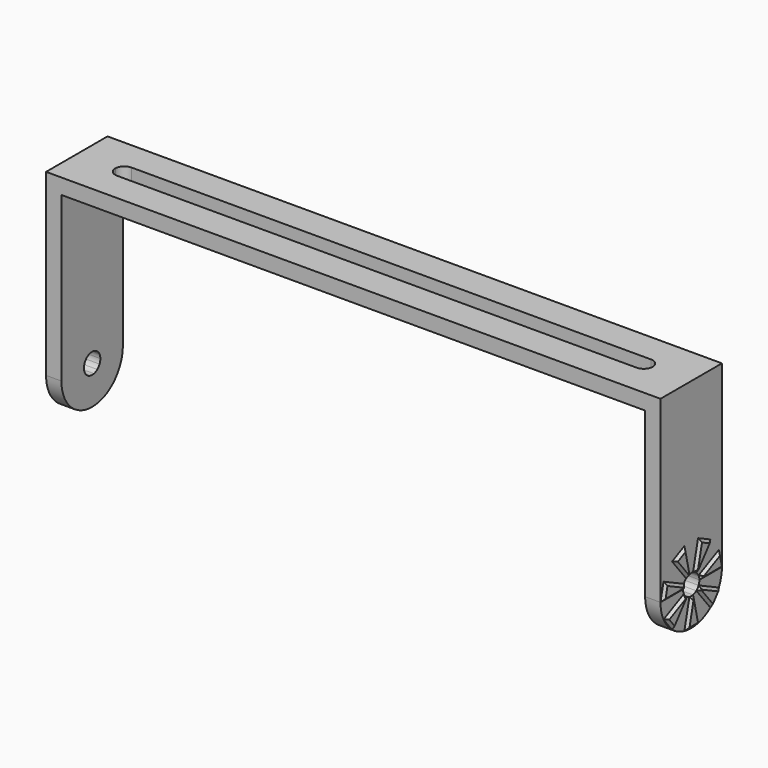
from build123d import *

# Parameters (mm, degrees)
F0_W                     = 3
F0_H                     = 15
F1_DEPTH                 = 35
F2_DEPTH                 = 3
F3_W                     = 3
F3_H                     = 7.5
F6_DEPTH                 = 0.5
DRAFT_F6_DRAFTED_ANGLE   = 45
DRAFT_F6_2_DRAFTED_ANGLE = 45
DRAFT_F6_3_DRAFTED_ANGLE = 45
DRAFT_F6_4_DRAFTED_ANGLE = 45
DRAFT_F6_5_DRAFTED_ANGLE = 45
DRAFT_F6_6_DRAFTED_ANGLE = 45
DRAFT_F6_7_DRAFTED_ANGLE = 45
F7_DEPTH                 = 25


# Not quite as in the source:
# - an extrude with a draft is written as a straight extrude whose walls are then drafted


with BuildPart() as f1:
    # F0 (on Top) → F1 (new body)
    with BuildSketch(Plane.XY):
        with Locations((-58.5, 0)):
            Rectangle(F0_W, F0_H)
    extrude(amount=-F1_DEPTH)

    # F0 (on Top) → F2 (join)
    with BuildSketch(Plane.XY):
        with BuildLine():
            Line((0, 1.75), (0, 7.5))
            Line((0, 7.5), (-57, 7.5))
            Line((-57, 7.5), (-57, -7.5))
            Line((-57, -7.5), (0, -7.5))
            Line((0, -7.5), (0, -1.75))
            Line((0, -1.75), (-50.7319065422, -1.75))
            ThreePointArc((-50.7319065422, -1.75), (-51.9693434093, -1.2374368671), (-52.4819065422, 0))
            ThreePointArc((-52.4819065422, 0), (-51.9693434093, 1.2374368671), (-50.7319065422, 1.75))
            Line((-50.7319065422, 1.75), (0, 1.75))
        make_face()
    extrude(amount=-F2_DEPTH)

    # F3 (on face) → F4 (revolve)
    with BuildSketch(Plane(origin=(0, 0, -35), x_dir=(1, 0, 0), z_dir=(0, 0, -1))):
        with Locations((-58.5, 3.75)):
            Rectangle(F3_W, F3_H)
    revolve(axis=Axis((-54.6439792961, 0, -35), (1, 0, 0)))


with BuildPart() as f6_drafted:
    # F5 (on face) → F6 (new body)
    with BuildSketch(Plane(origin=(-60, 0, 0), x_dir=(0, -1, 0), z_dir=(-1, 0, 0))):
        with BuildLine():
            Line((4.6761735139, -40.8637361185), (6.7572665093, -38.2541280434))
            Line((6.7572665093, -38.2541280434), (1.8019377358, -35.8677674782))
            ThreePointArc((1.8019377358, -35.8677674782), (1.5636629649, -36.2469796037), (1.2469796037, -36.5636629649))
            Line((1.2469796037, -36.5636629649), (4.6761735139, -40.8637361185))
        make_face()
    extrude(amount=F6_DEPTH)

    # draft_F6_drafted
    draft_f6_drafted_walls = [f6_drafted.faces().sort_by_distance(p)[0] for p in [
        (-60.3333333333, -1.5636629649, -36.2469796037),
        (-60.3333333333, -2.9615765588, -38.7136995417),
        (-60.3333333333, -5.7167200116, -39.5589320809),
        (-60.3333333333, -4.2796021225, -37.0609477608),
    ]]
    draft(draft_f6_drafted_walls, neutral_plane=Plane(origin=(-60, 0, 0), x_dir=(0, -1, 0), z_dir=(-1, 0, 0)), angle=DRAFT_F6_DRAFTED_ANGLE)


with BuildPart() as f1_1:
    add(f1.part)

    # join_F6_drafted: union F6_drafted
    add(f6_drafted.part)


with BuildPart() as f6_2_drafted:
    # F5 (on face) → F6, piece 2 (new body)
    with BuildSketch(Plane(origin=(-60, 0, 0), x_dir=(0, -1, 0), z_dir=(-1, 0, 0))):
        with BuildLine():
            Line((-1.6689070047, -42.3119593414), (1.6689070047, -42.3119593414))
            Line((1.6689070047, -42.3119593414), (0.4450418679, -36.9498558244))
            ThreePointArc((0.4450418679, -36.9498558244), (0, -37), (-0.4450418679, -36.9498558244))
            Line((-0.4450418679, -36.9498558244), (-1.6689070047, -42.3119593414))
        make_face()
    extrude(amount=F6_DEPTH)

    # draft_F6_2_drafted
    draft_f6_2_drafted_walls = [f6_2_drafted.faces().sort_by_distance(p)[0] for p in [
        (-60.3333333333, 0, -37),
        (-60.3333333333, 1.0569744363, -39.6309075829),
        (-60.3333333333, 0, -42.3119593414),
        (-60.3333333333, -1.0569744363, -39.6309075829),
    ]]
    draft(draft_f6_2_drafted_walls, neutral_plane=Plane(origin=(-60, 0, 0), x_dir=(0, -1, 0), z_dir=(-1, 0, 0)), angle=DRAFT_F6_2_DRAFTED_ANGLE)


with BuildPart() as f1_2:
    add(f1_1.part)

    # join_F6_2_drafted: union F6_2_drafted
    add(f6_2_drafted.part)


with BuildPart() as f6_3_drafted:
    # F5 (on face) → F6, piece 3 (new body)
    with BuildSketch(Plane(origin=(-60, 0, 0), x_dir=(0, -1, 0), z_dir=(-1, 0, 0))):
        with BuildLine():
            Line((-1.8019377358, -35.8677674782), (-6.7572665093, -38.2541280434))
            Line((-6.7572665093, -38.2541280434), (-4.6761735139, -40.8637361185))
            Line((-4.6761735139, -40.8637361185), (-1.2469796037, -36.5636629649))
            ThreePointArc((-1.2469796037, -36.5636629649), (-1.5636629649, -36.2469796037), (-1.8019377358, -35.8677674782))
        make_face()
    extrude(amount=F6_DEPTH)

    # draft_F6_3_drafted
    draft_f6_3_drafted_walls = [f6_3_drafted.faces().sort_by_distance(p)[0] for p in [
        (-60.3333333333, 2.9615765588, -38.7136995417),
        (-60.3333333333, 1.5636629649, -36.2469796037),
        (-60.3333333333, 4.2796021225, -37.0609477608),
        (-60.3333333333, 5.7167200116, -39.5589320809),
    ]]
    draft(draft_f6_3_drafted_walls, neutral_plane=Plane(origin=(-60, 0, 0), x_dir=(0, -1, 0), z_dir=(-1, 0, 0)), angle=DRAFT_F6_3_DRAFTED_ANGLE)


with BuildPart() as f1_3:
    add(f1_2.part)

    # join_F6_3_drafted: union F6_3_drafted
    add(f6_3_drafted.part)


with BuildPart() as f6_4_drafted:
    # F5 (on face) → F6, piece 4 (new body)
    with BuildSketch(Plane(origin=(-60, 0, 0), x_dir=(0, -1, 0), z_dir=(-1, 0, 0))):
        with BuildLine():
            Line((-6.7572665093, -31.7458719566), (-7.5, -35))
            Line((-7.5, -35), (-2, -35))
            ThreePointArc((-2, -35), (-1.9498558244, -34.5549581321), (-1.8019377358, -34.1322325218))
            Line((-1.8019377358, -34.1322325218), (-6.7572665093, -31.7458719566))
        make_face()
    extrude(amount=F6_DEPTH)

    # draft_F6_4_drafted
    draft_f6_4_drafted_walls = [f6_4_drafted.faces().sort_by_distance(p)[0] for p in [
        (-60.3333333333, 4.2796021225, -32.9390522392),
        (-60.3333333333, 7.1286332546, -33.3729359783),
        (-60.3333333333, 4.75, -35),
        (-60.3333333333, 1.9498558244, -34.5549581321),
    ]]
    draft(draft_f6_4_drafted_walls, neutral_plane=Plane(origin=(-60, 0, 0), x_dir=(0, -1, 0), z_dir=(-1, 0, 0)), angle=DRAFT_F6_4_DRAFTED_ANGLE)


with BuildPart() as f1_4:
    add(f1_3.part)

    # join_F6_4_drafted: union F6_4_drafted
    add(f6_4_drafted.part)


with BuildPart() as f6_5_drafted:
    # F5 (on face) → F6, piece 5 (new body)
    with BuildSketch(Plane(origin=(-60, 0, 0), x_dir=(0, -1, 0), z_dir=(-1, 0, 0))):
        with BuildLine():
            Line((-0.4450418679, -33.0501441756), (-1.6689070047, -27.6880406586))
            Line((-1.6689070047, -27.6880406586), (-4.6761735139, -29.1362638815))
            Line((-4.6761735139, -29.1362638815), (-1.2469796037, -33.4363370351))
            ThreePointArc((-1.2469796037, -33.4363370351), (-0.8677674782, -33.1980622642), (-0.4450418679, -33.0501441756))
        make_face()
    extrude(amount=F6_DEPTH)

    # draft_F6_5_drafted
    draft_f6_5_drafted_walls = [f6_5_drafted.faces().sort_by_distance(p)[0] for p in [
        (-60.3333333333, 0.8677674782, -33.1980622642),
        (-60.3333333333, 1.0569744363, -30.3690924171),
        (-60.3333333333, 3.1725402593, -28.4121522701),
        (-60.3333333333, 2.9615765588, -31.2863004583),
    ]]
    draft(draft_f6_5_drafted_walls, neutral_plane=Plane(origin=(-60, 0, 0), x_dir=(0, -1, 0), z_dir=(-1, 0, 0)), angle=DRAFT_F6_5_DRAFTED_ANGLE)


with BuildPart() as f1_5:
    add(f1_4.part)

    # join_F6_5_drafted: union F6_5_drafted
    add(f6_5_drafted.part)


with BuildPart() as f6_6_drafted:
    # F5 (on face) → F6, piece 6 (new body)
    with BuildSketch(Plane(origin=(-60, 0, 0), x_dir=(0, -1, 0), z_dir=(-1, 0, 0))):
        with BuildLine():
            Line((1.2469796037, -33.4363370351), (4.6761735139, -29.1362638815))
            Line((4.6761735139, -29.1362638815), (1.6689070047, -27.6880406586))
            Line((1.6689070047, -27.6880406586), (0.4450418679, -33.0501441756))
            ThreePointArc((0.4450418679, -33.0501441756), (0.8677674782, -33.1980622642), (1.2469796037, -33.4363370351))
        make_face()
    extrude(amount=F6_DEPTH)

    # draft_F6_6_drafted
    draft_f6_6_drafted_walls = [f6_6_drafted.faces().sort_by_distance(p)[0] for p in [
        (-60.3333333333, -1.0569744363, -30.3690924171),
        (-60.3333333333, -0.8677674782, -33.1980622642),
        (-60.3333333333, -2.9615765588, -31.2863004583),
        (-60.3333333333, -3.1725402593, -28.4121522701),
    ]]
    draft(draft_f6_6_drafted_walls, neutral_plane=Plane(origin=(-60, 0, 0), x_dir=(0, -1, 0), z_dir=(-1, 0, 0)), angle=DRAFT_F6_6_DRAFTED_ANGLE)


with BuildPart() as f1_6:
    add(f1_5.part)

    # join_F6_6_drafted: union F6_6_drafted
    add(f6_6_drafted.part)


with BuildPart() as f6_7_drafted:
    # F5 (on face) → F6, piece 7 (new body)
    with BuildSketch(Plane(origin=(-60, 0, 0), x_dir=(0, -1, 0), z_dir=(-1, 0, 0))):
        with BuildLine():
            Line((2, -35), (7.5, -35))
            Line((7.5, -35), (6.7572665093, -31.7458719566))
            Line((6.7572665093, -31.7458719566), (1.8019377358, -34.1322325218))
            ThreePointArc((1.8019377358, -34.1322325218), (1.9498558244, -34.5549581321), (2, -35))
        make_face()
    extrude(amount=F6_DEPTH)

    # draft_F6_7_drafted
    draft_f6_7_drafted_walls = [f6_7_drafted.faces().sort_by_distance(p)[0] for p in [
        (-60.3333333333, -1.9498558244, -34.5549581321),
        (-60.3333333333, -4.75, -35),
        (-60.3333333333, -7.1286332546, -33.3729359783),
        (-60.3333333333, -4.2796021225, -32.9390522392),
    ]]
    draft(draft_f6_7_drafted_walls, neutral_plane=Plane(origin=(-60, 0, 0), x_dir=(0, -1, 0), z_dir=(-1, 0, 0)), angle=DRAFT_F6_7_DRAFTED_ANGLE)


with BuildPart() as f1_7:
    add(f1_6.part)

    # join_F6_7_drafted: union F6_7_drafted
    add(f6_7_drafted.part)

    # F5 (on face) → F7 (cut)
    with BuildSketch(Plane(origin=(-60, 0, 0), x_dir=(0, -1, 0), z_dir=(-1, 0, 0))):
        with BuildLine():
            ThreePointArc((1.8019377358, -35.8677674782), (1.9498558244, -35.4450418679), (2, -35))
            ThreePointArc((2, -35), (1.9498558244, -34.5549581321), (1.8019377358, -34.1322325218))
            ThreePointArc((1.8019377358, -34.1322325218), (1.5636629649, -33.7530203963), (1.2469796037, -33.4363370351))
            ThreePointArc((1.2469796037, -33.4363370351), (0.8677674782, -33.1980622642), (0.4450418679, -33.0501441756))
            ThreePointArc((0.4450418679, -33.0501441756), (0, -33), (-0.4450418679, -33.0501441756))
            ThreePointArc((-0.4450418679, -33.0501441756), (-0.8677674782, -33.1980622642), (-1.2469796037, -33.4363370351))
            ThreePointArc((-1.2469796037, -33.4363370351), (-1.5636629649, -33.7530203963), (-1.8019377358, -34.1322325218))
            ThreePointArc((-1.8019377358, -34.1322325218), (-1.9498558244, -34.5549581321), (-2, -35))
            ThreePointArc((-2, -35), (-1.9498558244, -35.4450418679), (-1.8019377358, -35.8677674782))
            ThreePointArc((-1.8019377358, -35.8677674782), (-1.5636629649, -36.2469796037), (-1.2469796037, -36.5636629649))
            ThreePointArc((-1.2469796037, -36.5636629649), (-0.8677674782, -36.8019377358), (-0.4450418679, -36.9498558244))
            ThreePointArc((-0.4450418679, -36.9498558244), (0, -37), (0.4450418679, -36.9498558244))
            ThreePointArc((0.4450418679, -36.9498558244), (0.8677674782, -36.8019377358), (1.2469796037, -36.5636629649))
            ThreePointArc((1.2469796037, -36.5636629649), (1.5636629649, -36.2469796037), (1.8019377358, -35.8677674782))
        make_face()
    extrude(amount=-F7_DEPTH, mode=Mode.SUBTRACT)

    # F8: F1 across plane


with BuildPart() as f1_8:
    add(f1_7.part)
    add(f1_7.part.mirror(Plane.YZ))


solid = f1_8.part
